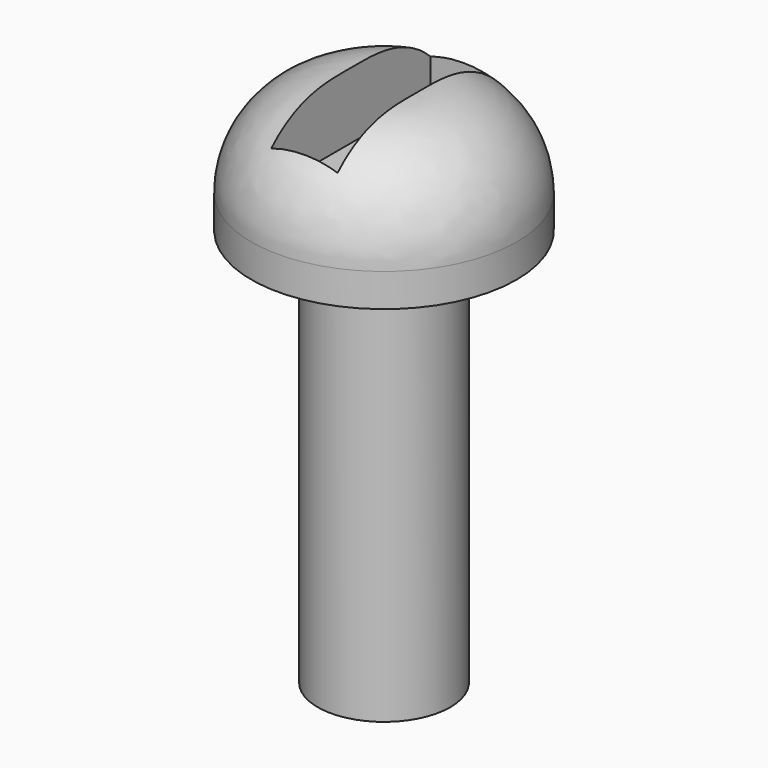
from build123d import *

# Parameters (mm, degrees)
F0_R     = 1.27
F1_DEPTH = 7.62
F2_R     = 2.54
F3_DEPTH = 2.54
F4_W     = 1.27
F4_H     = 3.81
F5_DEPTH = 1.27


# Not quite as in the source:
# - a fillet or chamfer that OpenCascade refuses, or shapes differently, is made with other operations: its cross-section is extruded or revolved along the edge and cut away or added


with BuildPart() as f1:
    # F0 (on Top) → F1 (new body)
    with BuildSketch(Plane.XY):
        Circle(F0_R)
    extrude(amount=F1_DEPTH)

    # F2 (on face) → F3 (join)
    with BuildSketch(Plane.XY.offset(7.62)):
        Circle(F2_R)
    extrude(amount=F3_DEPTH)

    # F4 (on face) → F5 (cut)
    with BuildSketch(Plane.XY.offset(10.16)):
        Rectangle(F4_W, F4_H)
    extrude(amount=-F5_DEPTH, mode=Mode.SUBTRACT)

    # F6: fillet of radius 1.905 on 1 edges, made by hand

    # F6_s1 → F6_t2 (revolve, cut)
    with BuildSketch(Plane.XZ):
        with BuildLine():
            ThreePointArc((2.54, 8.255), (1.9820384182, 9.6020384182), (0.635, 10.16))
            Line((0.635, 10.16), (2.54, 10.16))
            Line((2.54, 10.16), (2.54, 8.255))
        make_face()
    revolve(axis=Axis((0, 0, 10.16), (0, 0, 1)), mode=Mode.SUBTRACT)


solid = f1.part
